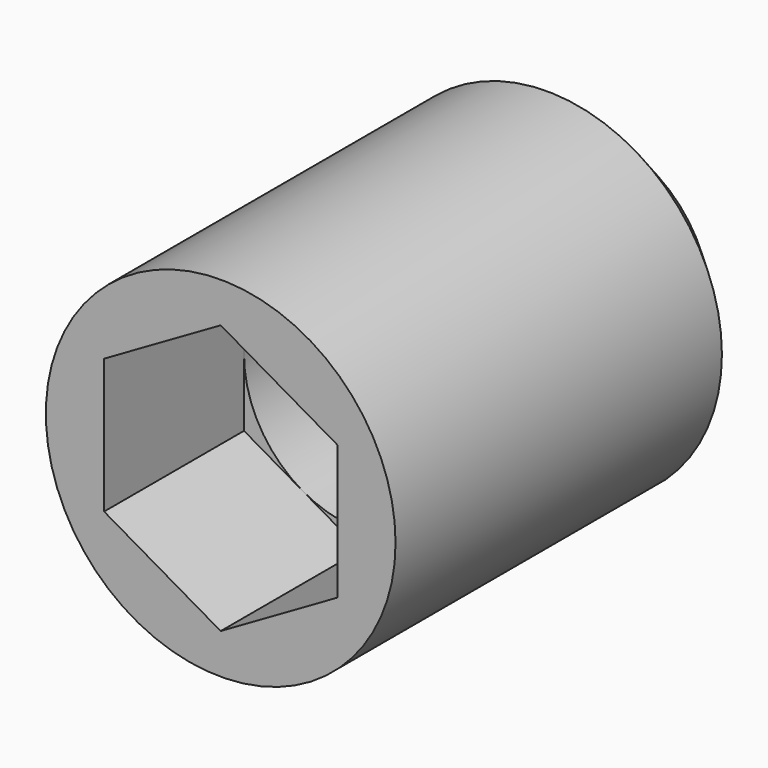
from build123d import *

# Parameters (mm, degrees)
F0_R     = 3
F1_DEPTH = 8
F3_DEPTH = 3
F4_R     = 2
F5_DEPTH = 25
F6_SIZE  = 0.99999


# Not quite as in the source:
# - a fillet or chamfer is up to 0.001 mm smaller than in the source, because OpenCascade refuses the exact size


with BuildPart() as f1:
    # F0 (on Front) → F1 (new body)
    with BuildSketch(Plane.XZ):
        Circle(F0_R)
    extrude(amount=F1_DEPTH)

    # F2 (on face) → F3 (cut)
    with BuildSketch(Plane.XZ.offset(8)):
        Polygon((2, 1.1547005384), (0, 2.3094010768), (-2, 1.1547005384), (-2, -1.1547005384), (0, -2.3094010768), (2, -1.1547005384), align=None)
    extrude(amount=-F3_DEPTH, mode=Mode.SUBTRACT)

    # F4 (on face) → F5 (cut)
    with BuildSketch(Plane.XZ.offset(5)):
        Circle(F4_R)
    extrude(amount=-F5_DEPTH, mode=Mode.SUBTRACT)

    # F6 (size 1 in the source; OpenCascade refuses exactly that, so slightly less here)
    f6_edges = [f1.edges().sort_by_distance(p)[0] for p in [
        (-3, 0, 0),
    ]]
    chamfer(f6_edges, length=F6_SIZE)


solid = f1.part
